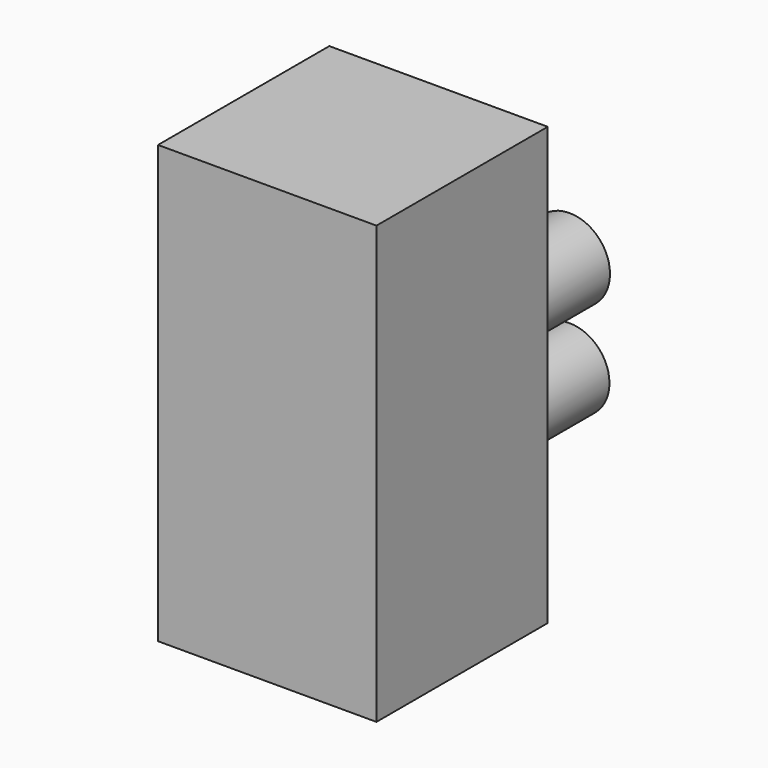
from build123d import *

# Parameters (mm, degrees)
F0_W     = 25.4
F0_H     = 50.8
F1_DEPTH = 24.892
F2_R     = 4.6961896277
F2_R_2   = 4.6352376904
F3_DEPTH = 19.05


# Not quite as in the source:
# - a feature names something its author has since deleted; it is built from what else it names


with BuildPart() as f1:
    # F0 (on Front) → F1 (new body)
    with BuildSketch(Plane.XZ):
        Rectangle(F0_W, F0_H)
    extrude(amount=F1_DEPTH)

    # F2 (on Front) → F3 (join)
    with BuildSketch(Plane.XZ):
        Circle(F2_R)
        with Locations((0, -11.2072117627)):
            Circle(F2_R_2)
    extrude(amount=-F3_DEPTH)


solid = f1.part
